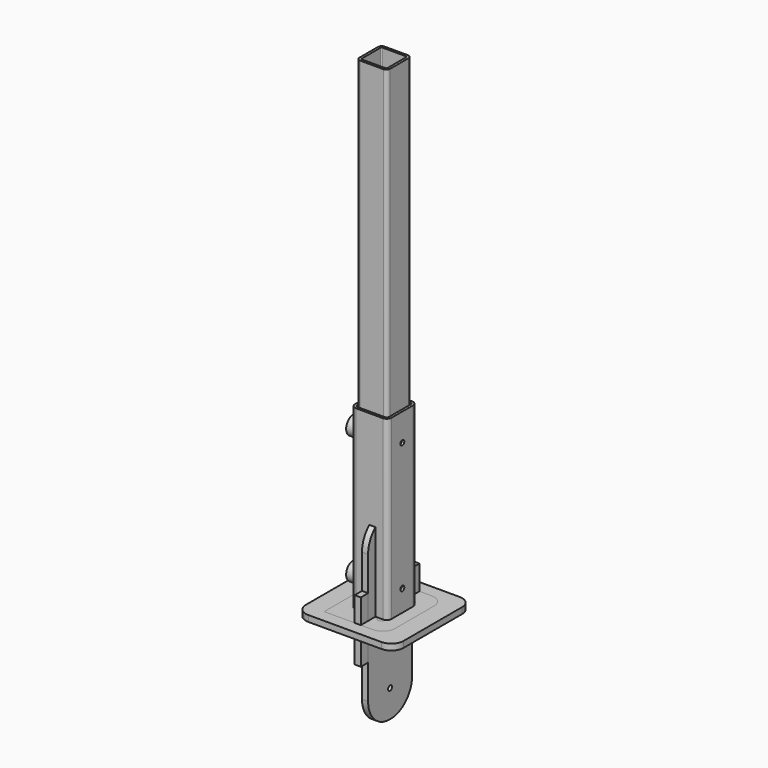
from build123d import *
from build123d import SkipClean  # not in build123d's __all__

# Parameters (mm, degrees)
F1_DEPTH  = 5
F2_W      = 60
F2_H      = 50
F3_DEPTH  = 5
F4_R      = 3
F5_DEPTH  = 5
F7_DEPTH  = 400
F9_DEPTH  = 150
F10_R     = 2
F11_DEPTH = 35
F12_R     = 7.5
F12_R_2   = 2
F13_DEPTH = 10
F14_R     = 2
F15_DEPTH = 5


with BuildPart() as f1:
    # F0 (on Top) → F1 (new body)
    with BuildSketch(Plane.XY):
        with BuildLine():
            ThreePointArc((-40, -30), (-37.0710678119, -37.0710678119), (-30, -40))
            Line((-30, -40), (30, -40))
            ThreePointArc((30, -40), (37.0710678119, -37.0710678119), (40, -30))
            Line((40, -30), (40, 30))
            ThreePointArc((40, 30), (37.0710678119, 37.0710678119), (30, 40))
            Line((30, 40), (-30, 40))
            ThreePointArc((-30, 40), (-37.0710678119, 37.0710678119), (-40, 30))
            Line((-40, 30), (-40, -30))
        make_face()
    extrude(amount=F1_DEPTH)


with BuildPart() as f3:
    # F2 (on Right) → F3 (new body)
    with BuildSketch(Plane.YZ):
        Rectangle(F2_W, F2_H)
    extrude(amount=F3_DEPTH)


with BuildPart() as f5:
    # F4 (on Top) → F5 (new body)
    with BuildSketch(Plane.XY):
        with BuildLine():
            ThreePointArc((25, 20), (22.0710678119, 27.0710678119), (15, 30))
            Line((15, 30), (-25, 30))
            Line((-25, 30), (-25, -30))
            Line((-25, -30), (15, -30))
            ThreePointArc((15, -30), (22.0710678119, -27.0710678119), (25, -20))
            Line((25, -20), (25, 20))
        make_face()
        with Locations((10, -15)):
            Circle(F4_R, mode=Mode.SUBTRACT)
        with Locations((10, 15)):
            Circle(F4_R, mode=Mode.SUBTRACT)
    extrude(amount=F5_DEPTH)


with BuildPart() as f7:
    # F6 (on Top) → F7 (new body)
    with BuildSketch(Plane.XY):
        with BuildLine():
            ThreePointArc((12.5, 9.5), (11.6213203436, 11.6213203436), (9.5, 12.5))
            Line((9.5, 12.5), (-9.5, 12.5))
            ThreePointArc((-9.5, 12.5), (-11.6213203436, 11.6213203436), (-12.5, 9.5))
            Line((-12.5, 9.5), (-12.5, -9.5))
            ThreePointArc((-12.5, -9.5), (-11.6213203436, -11.6213203436), (-9.5, -12.5))
            Line((-9.5, -12.5), (9.5, -12.5))
            ThreePointArc((9.5, -12.5), (11.6213203436, -11.6213203436), (12.5, -9.5))
            Line((12.5, -9.5), (12.5, 9.5))
        make_face()
        with BuildLine():
            ThreePointArc((9.5, 10.5), (10.2071067812, 10.2071067812), (10.5, 9.5))
            Line((10.5, 9.5), (10.5, -9.5))
            ThreePointArc((10.5, -9.5), (10.2071067812, -10.2071067812), (9.5, -10.5))
            Line((9.5, -10.5), (-9.5, -10.5))
            ThreePointArc((-9.5, -10.5), (-10.2071067812, -10.2071067812), (-10.5, -9.5))
            Line((-10.5, -9.5), (-10.5, 9.5))
            ThreePointArc((-10.5, 9.5), (-10.2071067812, 10.2071067812), (-9.5, 10.5))
            Line((-9.5, 10.5), (9.5, 10.5))
        make_face(mode=Mode.SUBTRACT)
    extrude(amount=F7_DEPTH)


with BuildPart() as f9:
    # F8 (on Top) → F9 (new body)
    with BuildSketch(Plane.XY):
        with BuildLine():
            ThreePointArc((15, 11), (13.8284271247, 13.8284271247), (11, 15))
            Line((11, 15), (-11, 15))
            ThreePointArc((-11, 15), (-13.8284271247, 13.8284271247), (-15, 11))
            Line((-15, 11), (-15, -11))
            ThreePointArc((-15, -11), (-13.8284271247, -13.8284271247), (-11, -15))
            Line((-11, -15), (11, -15))
            ThreePointArc((11, -15), (13.8284271247, -13.8284271247), (15, -11))
            Line((15, -11), (15, 11))
        make_face()
        with BuildLine():
            ThreePointArc((11, 13), (12.4142135624, 12.4142135624), (13, 11))
            Line((13, 11), (13, -11))
            ThreePointArc((13, -11), (12.4142135624, -12.4142135624), (11, -13))
            Line((11, -13), (-11, -13))
            ThreePointArc((-11, -13), (-12.4142135624, -12.4142135624), (-13, -11))
            Line((-13, -11), (-13, 11))
            ThreePointArc((-13, 11), (-12.4142135624, 12.4142135624), (-11, 13))
            Line((-11, 13), (11, 13))
        make_face(mode=Mode.SUBTRACT)
    extrude(amount=F9_DEPTH)

    # F10 (on face) → F11 (cut)
    with BuildSketch(Plane.YZ.offset(15)):
        with Locations((0, 127.5)):
            Circle(F10_R)
        with Locations((0, 22.5)):
            Circle(F10_R)
    extrude(amount=-F11_DEPTH, mode=Mode.SUBTRACT)

    # F12 (on face) → F13 (join)
    with BuildSketch(Plane(origin=(-15, 0, 0), x_dir=(0, -1, 0), z_dir=(-1, 0, 0))):
        with Locations((0, 127.5)):
            Circle(F12_R)
        with Locations((0, 127.5)):
            Circle(F12_R_2, mode=Mode.SUBTRACT)
        with Locations((0, 22.5)):
            Circle(F12_R)
        with Locations((0, 22.5)):
            Circle(F12_R_2, mode=Mode.SUBTRACT)
    with SkipClean():  # cleaning this boolean's faces spoils the solid; the shape is the same uncleaned
        extrude(amount=F13_DEPTH)


with BuildPart() as f15:
    # F14 (on Right) → F15 (new body)
    with BuildSketch(Plane.YZ):
        with BuildLine():
            ThreePointArc((-22.5, -53), (-16.0563491861, -68.5563491861), (-0.5, -75))
            Line((-0.5, -75), (0.5, -75))
            ThreePointArc((0.5, -75), (16.0563491861, -68.5563491861), (22.5, -53))
            Line((22.5, -53), (22.5, 53))
            ThreePointArc((22.5, 53), (16.0563491861, 68.5563491861), (0.5, 75))
            Line((0.5, 75), (-0.5, 75))
            ThreePointArc((-0.5, 75), (-16.0563491861, 68.5563491861), (-22.5, 53))
            Line((-22.5, 53), (-22.5, -53))
        make_face()
        with Locations((0, -52.5)):
            Circle(F14_R, mode=Mode.SUBTRACT)
        with Locations((0, 52.5)):
            Circle(F14_R, mode=Mode.SUBTRACT)
    extrude(amount=F15_DEPTH)


solid = Compound([f1.part, f3.part, f5.part, f7.part, f9.part, f15.part])
